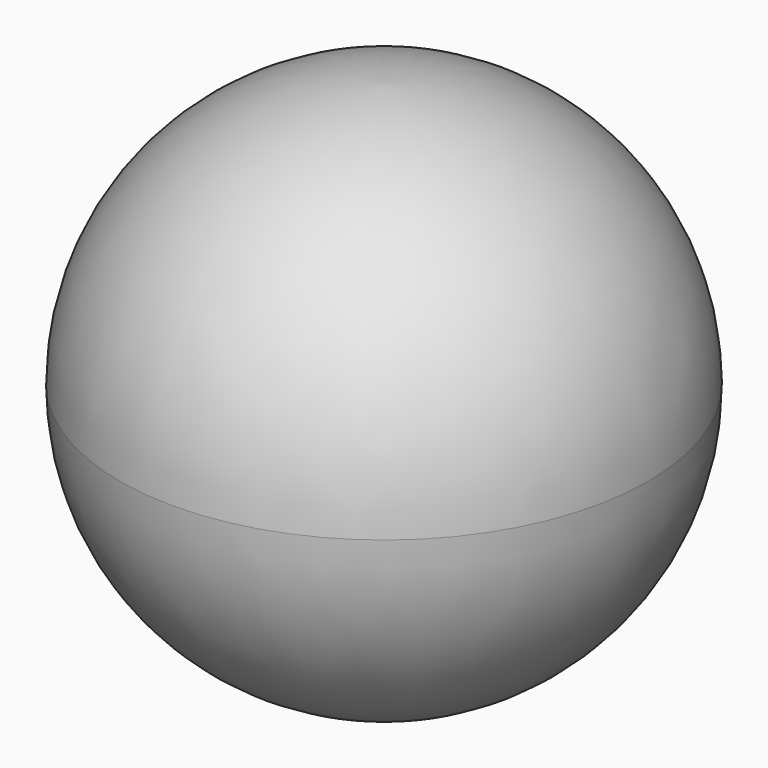
from build123d import *

# Parameters (mm, degrees)
F0_R     = 30
F1_DEPTH = 60
F2_R     = 29.99999


# Not quite as in the source:
# - a fillet or chamfer is up to 0.001 mm smaller than in the source, because OpenCascade refuses the exact size


with BuildPart() as f1:
    # F0 (on Top) → F1 (new body)
    with BuildSketch(Plane.XY):
        Circle(F0_R)
    extrude(amount=F1_DEPTH)

    # F2 (radius 30 in the source; OpenCascade refuses exactly that, so slightly less here)
    f2_edges = [f1.edges().sort_by_distance(p)[0] for p in [
        (-30, 0, 0),
        (-30, 0, 60),
    ]]
    fillet(f2_edges, radius=F2_R)


solid = f1.part
